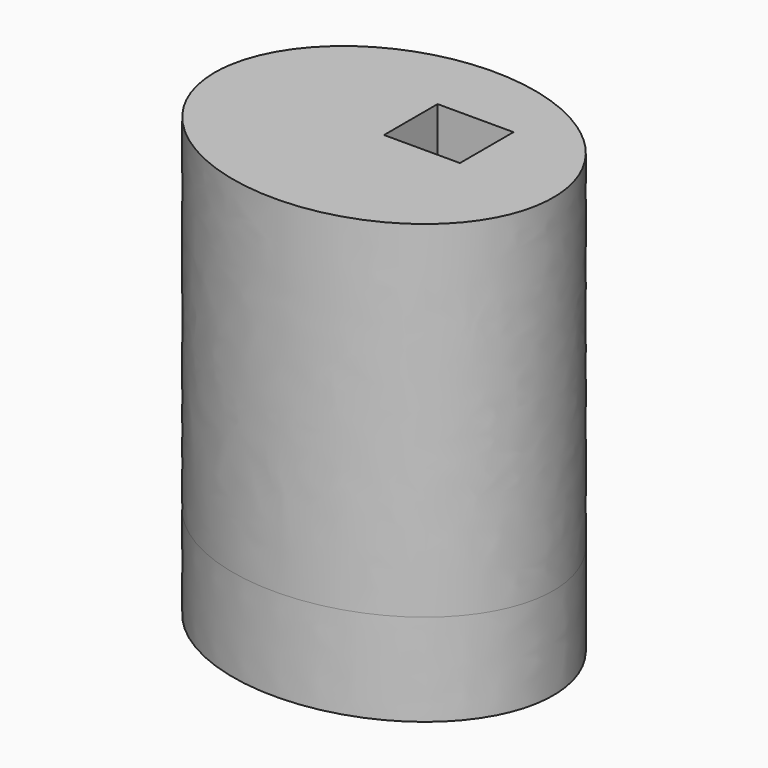
from build123d import *

# Parameters (mm, degrees)
F1_DEPTH = 25
F2_W     = 20.5906555057
F2_H     = 18.1680545211
F3_DEPTH = 25
F6_DEPTH = 93.8682109118


# Not quite as in the source:
# - the program builds the solid bodies; features that only make, move or delete a surface that nothing else refers to are left out


with BuildPart() as f1:
    # F0 (on Top) → F1 (new body)
    with BuildSketch(Plane.XY):
        with BuildLine():
            add(Edge.make_bspline(
                [(-22.398095578, 26.1815339327), (-22.398095578, -38.287113302), (46.4851502329, -6.0527896847), (115.3683960438, 26.1815339327), (46.4851502329, 58.41585755), (-22.398095578, 90.6501811674), (-22.398095578, 26.1815339327)],
                knots=[0, 0, 0, 2.0943951024, 2.0943951024, 4.1887902048, 4.1887902048, 6.2831853072, 6.2831853072, 6.2831853072], degree=2, weights=[1, 0.5, 1, 0.5, 1, 0.5, 1]))
        make_face()
    extrude(amount=F1_DEPTH)

    # F2 (on face) → F3 (join)
    with BuildSketch(Plane.XY.offset(25)):
        with Locations((33.8193960488, 35.2655611932)):
            Rectangle(F2_W, F2_H)
    extrude(amount=F3_DEPTH)

    # F6 (add): a face of the model
    f6_faces = [f1.faces().sort_by_distance(p)[0] for p in [
        (22.6964116523, 25.5040831256, 25),
    ]]
    extrude(f6_faces, amount=F6_DEPTH)


solid = f1.part
